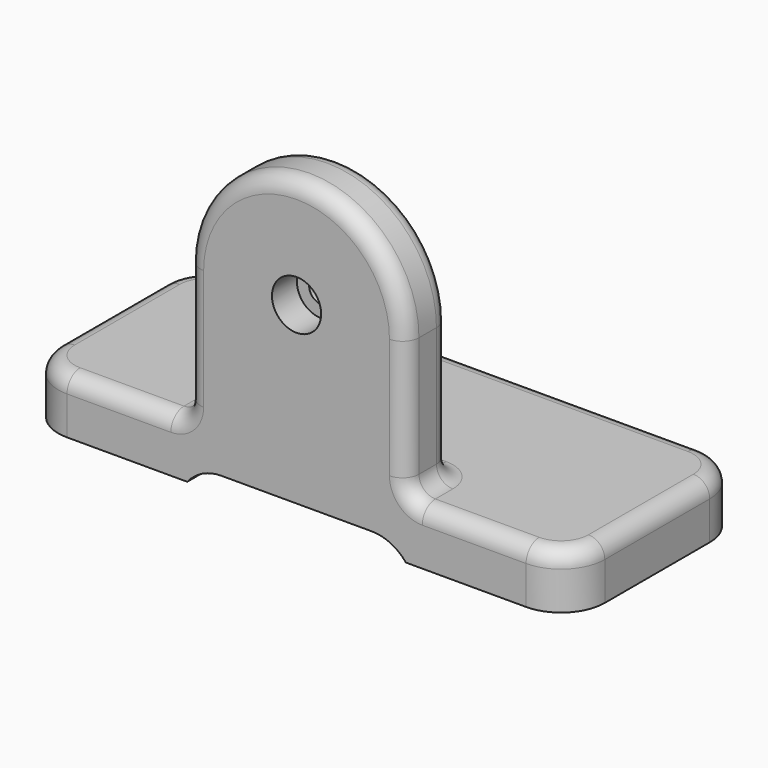
from build123d import *

# Parameters (mm, degrees)
F0_W          = 100
F0_H          = 40
F1_DEPTH      = 10
F3_DEPTH      = 10
F4_W          = 40
F4_H          = 3
F5_DEPTH      = 40.001
F6_R          = 2.25
F7_DEPTH      = 5.7
F8_R          = 2.25
F9_DEPTH      = 40.001
F10_R         = 4.5
F11_DEPTH     = 5.7
F12_T1_DEPTH  = 40
F12_T3_DEPTH  = 40
F12_T5_DEPTH  = 50
F12_T7_DEPTH  = 50
F12_T9_DEPTH  = 50
F12_T11_DEPTH = 50
F13_F1_R      = 3
F13_F2_R      = 3
F13_F3_R      = 3


# Not quite as in the source:
# - a fillet or chamfer that OpenCascade refuses, or shapes differently, is made with other operations: its cross-section is extruded or revolved along the edge and cut away or added


with BuildPart() as f1:
    # F0 (on Top) → F1 (new body)
    with BuildSketch(Plane.XY):
        with Locations((-50, 20)):
            Rectangle(F0_W, F0_H)
    extrude(amount=F1_DEPTH)

    # F2 (on Front) → F3 (join)
    with BuildSketch(Plane.XZ):
        with BuildLine():
            Line((-70, 35), (-70, 0))
            Line((-70, 0), (-30, 0))
            Line((-30, 0), (-30, 35))
            ThreePointArc((-30, 35), (-50, 55), (-70, 35))
        make_face()
    extrude(amount=-F3_DEPTH)

    # F4 (on face) → F5 (cut, through all)
    with BuildSketch(Plane.XZ):
        with Locations((-50, 1.5)):
            Rectangle(F4_W, F4_H)
    extrude(amount=-F5_DEPTH, mode=Mode.SUBTRACT)

    # F6 (on face) → F7 (cut)
    with BuildSketch(Plane.XZ):
        with Locations((-50, 35)):
            Circle(F6_R)
    extrude(amount=F7_DEPTH, mode=Mode.SUBTRACT)

    # F8 (on face) → F9 (cut, through all)
    with BuildSketch(Plane.XZ):
        with Locations((-50, 35)):
            Circle(F8_R)
    extrude(amount=-F9_DEPTH, mode=Mode.SUBTRACT)

    # F10 (on face) → F11 (cut)
    with BuildSketch(Plane.XZ):
        with Locations((-50, 35)):
            Circle(F10_R)
    extrude(amount=-F11_DEPTH, mode=Mode.SUBTRACT)

    # F12: fillet of radius 8 on 6 edges, made by hand

    # F12_s2 → F12_t1 (join)
    with BuildSketch(Plane.XZ.offset(-40)):
        with BuildLine():
            ThreePointArc((-70, 0), (-67.2191036167, 2.2111025509), (-63.7550020016, 3))
            Line((-63.7550020016, 3), (-70, 3))
            Line((-70, 3), (-70, 0))
        make_face()
    extrude(amount=F12_T1_DEPTH)

    # F12_s4 → F12_t3 (join)
    with BuildSketch(Plane.XZ.offset(-40)):
        with BuildLine():
            ThreePointArc((-36.2449979984, 3), (-32.7808963833, 2.2111025509), (-30, 0))
            Line((-30, 0), (-30, 3))
            Line((-30, 3), (-36.2449979984, 3))
        make_face()
    extrude(amount=F12_T3_DEPTH)

    # F12_s6 → F12_t5 (cut)
    with BuildSketch(Plane.XY.offset(-20)):
        with BuildLine():
            ThreePointArc((-92, 0), (-97.6568542495, 2.3431457505), (-100, 8))
            Line((-100, 8), (-100, 0))
            Line((-100, 0), (-92, 0))
        make_face()
    extrude(amount=F12_T5_DEPTH, mode=Mode.SUBTRACT)

    # F12_s8 → F12_t7 (cut)
    with BuildSketch(Plane.XY.offset(-20)):
        with BuildLine():
            ThreePointArc((-8, 0), (-2.3431457505, 2.3431457505), (0, 8))
            Line((0, 8), (0, 0))
            Line((0, 0), (-8, 0))
        make_face()
    extrude(amount=F12_T7_DEPTH, mode=Mode.SUBTRACT)

    # F12_s10 → F12_t9 (cut)
    with BuildSketch(Plane.XY.offset(-20)):
        with BuildLine():
            ThreePointArc((-100, 32), (-97.6568542495, 37.6568542495), (-92, 40))
            Line((-92, 40), (-100, 40))
            Line((-100, 40), (-100, 32))
        make_face()
    extrude(amount=F12_T9_DEPTH, mode=Mode.SUBTRACT)

    # F12_s12 → F12_t11 (cut)
    with BuildSketch(Plane.XY.offset(-20)):
        with BuildLine():
            ThreePointArc((-8, 40), (-2.3431457505, 37.6568542495), (0, 32))
            Line((0, 32), (0, 40))
            Line((0, 40), (-8, 40))
        make_face()
    extrude(amount=F12_T11_DEPTH, mode=Mode.SUBTRACT)

    # F13: fillet of radius 3 on 19 edges, made by hand

    # F13_f1
    f13_f1_edges = [f1.edges().sort_by_distance(p)[0] for p in [
        (-50, 10, 55),
        (-30, 10, 22.5),
        (-70, 10, 22.5),
    ]]
    fillet(f13_f1_edges, radius=F13_F1_R)

    # F13_f2
    f13_f2_edges = [f1.edges().sort_by_distance(p)[0] for p in [
        (-30, 3.5, 10),
        (-50, 10, 10),
        (-69.1213203436, 9.1213203436, 10),
        (-30.8786796564, 9.1213203436, 10),
    ]]
    fillet(f13_f2_edges, radius=F13_F2_R)

    # F13_f3
    f13_f3_edges = [f1.edges().sort_by_distance(p)[0] for p in [
        (-50, 0, 55),
        (-17.5, 0, 10),
        (-30, 0, 24),
        (-70, 0, 24),
        (-82.5, 0, 10),
        (-2.3431457505, 2.3431457505, 10),
        (-97.6568542495, 2.3431457505, 10),
        (-100, 20, 10),
        (-97.6568542495, 37.6568542495, 10),
        (-50, 40, 10),
        (-2.3431457505, 37.6568542495, 10),
        (0, 20, 10),
        (-70.8786796564, 0, 10.8786796564),
        (-29.1213203436, 0, 10.8786796564),
    ]]
    fillet(f13_f3_edges, radius=F13_F3_R)


solid = f1.part
